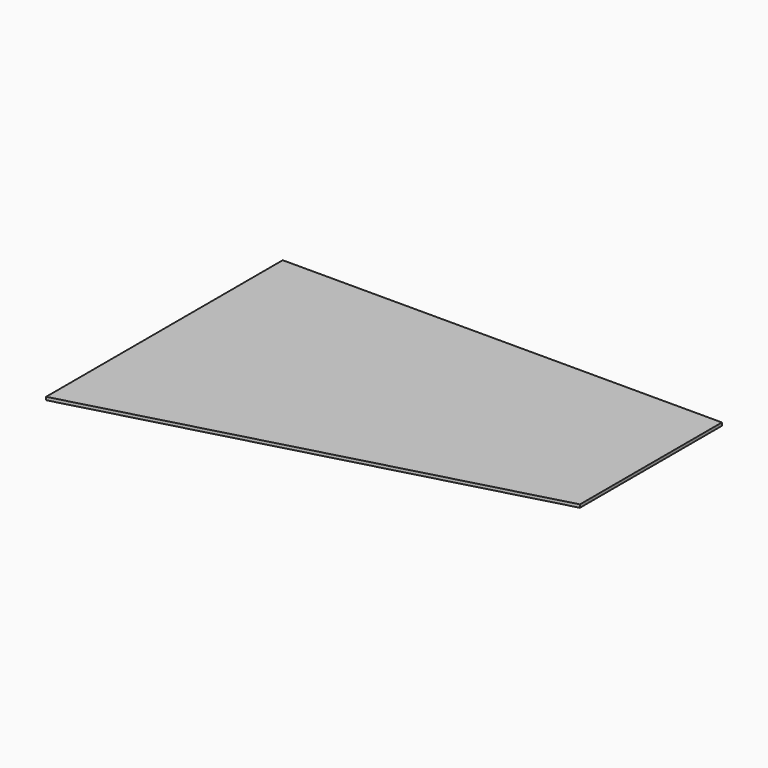
from build123d import *

# Parameters (mm, degrees)
F0_W     = 15
F0_H     = 3
F1_DEPTH = 3


with BuildPart() as f1:
    # F0 (on Top) → F1 (new body)
    with BuildSketch(Plane.XY):
        Polygon((252.2106605172, 212.4578239818), (-185.7893394828, 212.4578239818), (-185.7893394828, -82.5421760182), (252.2106605172, 35.4578239818), align=None)
        with Locations((-140.7893394828, 145.9578239818)):
            Rectangle(F0_W, F0_H, mode=Mode.SUBTRACT)
        with Locations((33.2106605172, 145.9578239818)):
            Rectangle(F0_W, F0_H, mode=Mode.SUBTRACT)
        with Locations((207.2106605172, 145.9578239818)):
            Rectangle(F0_W, F0_H, mode=Mode.SUBTRACT)
        with Locations((207.2106605172, 145.9578239818)):
            Rectangle(F0_W, F0_H)
        with Locations((-140.7893394828, 145.9578239818)):
            Rectangle(F0_W, F0_H)
        with Locations((33.2106605172, 145.9578239818)):
            Rectangle(F0_W, F0_H)
    extrude(amount=F1_DEPTH)


solid = f1.part
